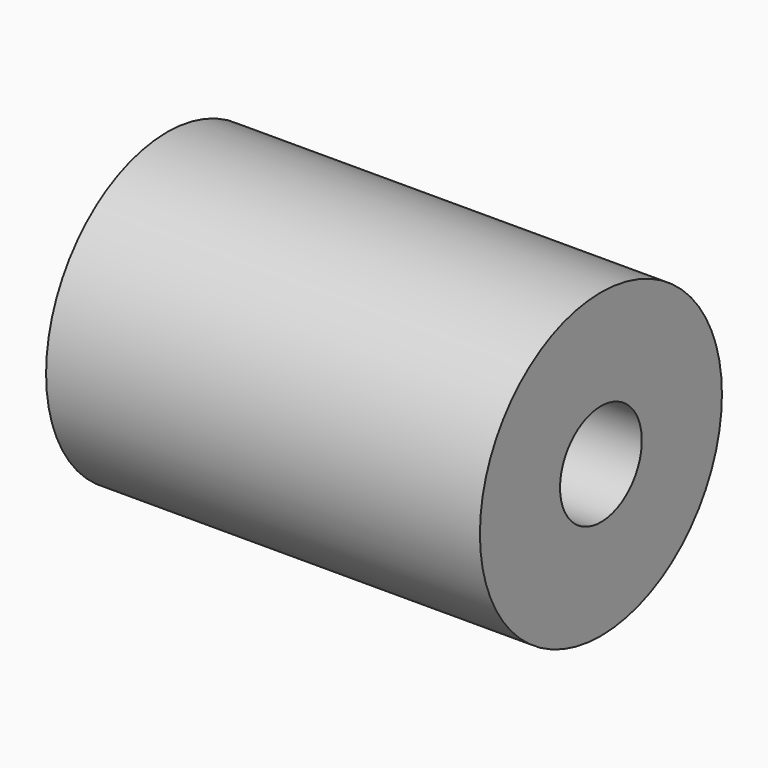
from build123d import *

# Parameters (mm, degrees)
F0_R     = 31.7020637967
F1_DEPTH = 90.932
F3_D     = 21.43125


# Not quite as in the source:
# - a length typed as a fraction of an inch, garbled in the dataset ("3 / 203.2 mm" for 3/8 in), is restored


with BuildPart() as f1:
    # F0 (on Right) → F1 (new body)
    with BuildSketch(Plane.YZ):
        with Locations((-73.6340805888, 47.5504361093)):
            Circle(F0_R)
    extrude(amount=F1_DEPTH)

    # F3 (through all)
    with Locations(Plane.YZ.offset(90.932)):
        with Locations((-73.6340805888, 47.5504361093)):
            Hole(F3_D / 2)


solid = f1.part
